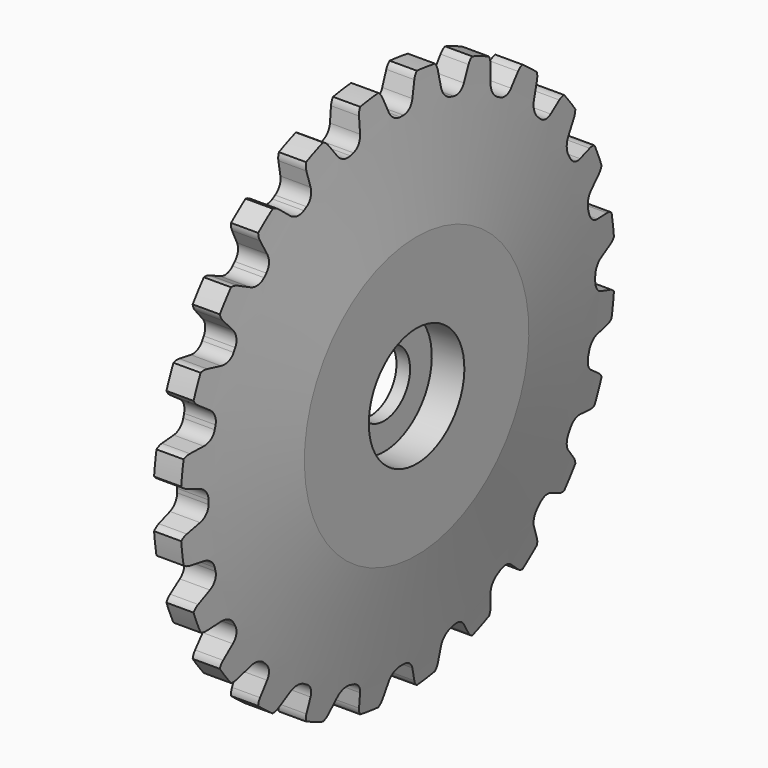
from build123d import *

# Parameters (mm, degrees)
F3_DEPTH        = 25
F4_DEPTH        = 25
F4_COPIES_COUNT = 24


# Not quite as in the source:
# - a feature of the source that left no trace in its solid (it failed there, or was rolled back) is left out
# - a pattern or mirror of a feature is missing from the dataset's text; its kind, count and spacing are read off the source's solid


with BuildPart() as f1:
    # F0 (on Front) → F1 (revolve)
    with BuildSketch(Plane.XZ):
        Polygon((0, 100), (0, 12), (5, 12), (5, 22), (17, 22), (17, 51.679217589), (10, 100), align=None)
    revolve(axis=Axis((6.5836515278, 0, 0), (1, 0, 0)))

    # F2 (on Right) → F3 (cut)
    with BuildSketch(Plane.YZ):
        with BuildLine():
            Line((-0.739408795, 89.0115863389), (0, 89.0115863389))
            Line((0, 89.0115863389), (0, 104.0115863389))
            Line((0, 104.0115863389), (-9.7, 104.0115863389))
            Line((-9.7, 104.0115863389), (-10.6611262397, 100.699401478))
            Line((-10.6611262397, 100.699401478), (-9.5657828926, 100.0876399393))
            ThreePointArc((-9.5657828926, 100.0876399393), (-8.1966159568, 98.9634782528), (-7.3053875823, 97.4324427928))
            Line((-7.3053875823, 97.4324427928), (-5.4378718989, 92.3014856223))
            ThreePointArc((-5.4378718989, 92.3014856223), (-3.6072909767, 89.9158261175), (-0.739408795, 89.0115863389))
        make_face()
        with BuildLine():
            Line((0, 104.0115863389), (0, 89.0115863389))
            Line((0, 89.0115863389), (0.739408795, 89.0115863389))
            ThreePointArc((0.739408795, 89.0115863389), (3.6072909767, 89.9158261175), (5.4378718989, 92.3014856223))
            Line((5.4378718989, 92.3014856223), (7.3053875823, 97.4324427928))
            ThreePointArc((7.3053875823, 97.4324427928), (8.1966159568, 98.9634782528), (9.5657828926, 100.0876399393))
            Line((9.5657828926, 100.0876399393), (10.6611262397, 100.699401478))
            Line((10.6611262397, 100.699401478), (9.7, 104.0115863389))
            Line((9.7, 104.0115863389), (0, 104.0115863389))
        make_face()
    extrude(amount=-F3_DEPTH, mode=Mode.SUBTRACT)

    # F2 (on Right) → F4 (cut)
    with BuildSketch(Plane.YZ):
        with BuildLine():
            Line((-0.739408795, 89.0115863389), (0, 89.0115863389))
            Line((0, 89.0115863389), (0, 104.0115863389))
            Line((0, 104.0115863389), (-9.7, 104.0115863389))
            Line((-9.7, 104.0115863389), (-10.6611262397, 100.699401478))
            Line((-10.6611262397, 100.699401478), (-9.5657828926, 100.0876399393))
            ThreePointArc((-9.5657828926, 100.0876399393), (-8.1966159568, 98.9634782528), (-7.3053875823, 97.4324427928))
            Line((-7.3053875823, 97.4324427928), (-5.4378718989, 92.3014856223))
            ThreePointArc((-5.4378718989, 92.3014856223), (-3.6072909767, 89.9158261175), (-0.739408795, 89.0115863389))
        make_face()
        with BuildLine():
            Line((0, 104.0115863389), (0, 89.0115863389))
            Line((0, 89.0115863389), (0.739408795, 89.0115863389))
            ThreePointArc((0.739408795, 89.0115863389), (3.6072909767, 89.9158261175), (5.4378718989, 92.3014856223))
            Line((5.4378718989, 92.3014856223), (7.3053875823, 97.4324427928))
            ThreePointArc((7.3053875823, 97.4324427928), (8.1966159568, 98.9634782528), (9.5657828926, 100.0876399393))
            Line((9.5657828926, 100.0876399393), (10.6611262397, 100.699401478))
            Line((10.6611262397, 100.699401478), (9.7, 104.0115863389))
            Line((9.7, 104.0115863389), (0, 104.0115863389))
        make_face()
    f4 = extrude(amount=F4_DEPTH, mode=Mode.SUBTRACT)

    # F4_copies: F4 ×24 about axis
    f4_copies_axis = Axis((0, 0, 0), (1, 0, 0))
    for i in range(1, F4_COPIES_COUNT):
        add(f4.rotate(f4_copies_axis, i * 360 / F4_COPIES_COUNT), mode=Mode.SUBTRACT)


solid = f1.part
